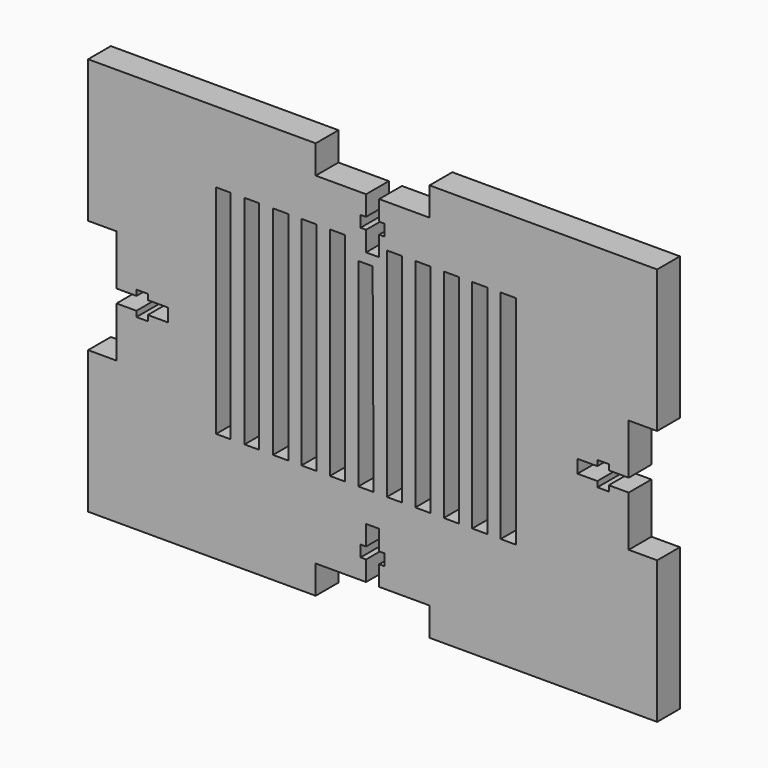
from build123d import *

# Parameters (mm, degrees)
F0_W     = 3.175
F0_H     = 48.4495080546
F0_W_2   = 3.4043772995
F1_DEPTH = 6.35


# Not quite as in the source:
# - a feature names something its author has since deleted; it is built from what else it names


with BuildPart() as f1:
    # F0 (on Front) → F1 (new body)
    with BuildSketch(Plane.XZ):
        Polygon((12.7, -44.45), (57.1500004709, -44.45), (63.5, -44.45), (63.5, -12.7), (57.1500004709, -12.7), (57.1500004709, -1.4605), (52.7050002354, -1.4605), (52.7050002354, -2.69367), (50.1650002354, -2.69367), (50.1650002354, -1.4605), (45.72, -1.4605), (45.72, 1.4605), (50.1650002354, 1.4605), (50.1650002354, 2.69367), (52.7050002354, 2.69367), (52.7050002354, 1.4605), (57.1500004709, 1.4605), (57.1500004709, 12.7), (63.5, 12.7), (63.5, 44.45), (57.1500004709, 44.45), (12.7, 44.45), (12.7, 38.1000004709), (1.4605, 38.1000004709), (1.4605, 33.6550002354), (2.69367, 33.6550002354), (2.69367, 31.1150002354), (1.4605, 31.1150002354), (1.4605, 26.67), (-1.4605, 26.67), (-1.4605, 31.1150002354), (-2.69367, 31.1150002354), (-2.69367, 33.6550002354), (-1.4605, 33.6550002354), (-1.4605, 38.1000004709), (-12.7, 38.1000004709), (-12.7, 44.45), (-57.1500004709, 44.45), (-63.5, 44.45), (-63.5, 12.7), (-57.1500004709, 12.7), (-57.1500004709, 1.4605), (-52.7050002354, 1.4605), (-52.7050002354, 2.69367), (-50.1650002354, 2.69367), (-50.1650002354, 1.4605), (-45.72, 1.4605), (-45.72, -1.4605), (-50.1650002354, -1.4605), (-50.1650002354, -2.69367), (-52.7050002354, -2.69367), (-52.7050002354, -1.4605), (-57.1500004709, -1.4605), (-57.1500004709, -2.69367), (-57.1500004709, -12.7), (-63.5, -12.7), (-63.5, -44.45), (-57.1500004709, -44.45), (-12.7, -44.45), (-12.7, -38.1000004709), (-1.4605, -38.1000004709), (-1.4605, -33.6550002354), (-2.69367, -33.6550002354), (-2.69367, -31.1150002354), (-1.4605, -31.1150002354), (-1.4605, -26.67), (1.4605, -26.67), (1.4605, -31.1150002354), (2.69367, -31.1150002354), (2.69367, -33.6550002354), (1.4605, -33.6550002354), (1.4605, -38.1000004709), (12.7, -38.1000004709), align=None)
        with Locations((-33.3375002354, 4.3502459727)):
            Rectangle(F0_W, F0_H, mode=Mode.SUBTRACT)
        with Locations((-26.9875002354, 4.3502459727)):
            Rectangle(F0_W, F0_H, mode=Mode.SUBTRACT)
        with Locations((-20.5228115857, 4.3502459727)):
            Rectangle(F0_W_2, F0_H, mode=Mode.SUBTRACT)
        with Locations((-14.1728115857, 4.3502459727)):
            Rectangle(F0_W_2, F0_H, mode=Mode.SUBTRACT)
        Polygon((0.2293770641, -19.8745080546), (-3.1750002354, -19.8745080546), (-3.1750002354, 24.4311112911), (0, 24.4311112911), align=None, mode=Mode.SUBTRACT)
        with Locations((-7.8228115857, 4.3502459727)):
            Rectangle(F0_W_2, F0_H, mode=Mode.SUBTRACT)
        with Locations((4.8771884143, 4.3502459727)):
            Rectangle(F0_W_2, F0_H, mode=Mode.SUBTRACT)
        with Locations((11.2271884143, 4.3502459727)):
            Rectangle(F0_W_2, F0_H, mode=Mode.SUBTRACT)
        with Locations((17.5771884143, 4.3502459727)):
            Rectangle(F0_W_2, F0_H, mode=Mode.SUBTRACT)
        with Locations((23.9271884143, 4.3502459727)):
            Rectangle(F0_W_2, F0_H, mode=Mode.SUBTRACT)
        with Locations((30.2771884143, 4.3502459727)):
            Rectangle(F0_W_2, F0_H, mode=Mode.SUBTRACT)
    extrude(amount=F1_DEPTH)


solid = f1.part
